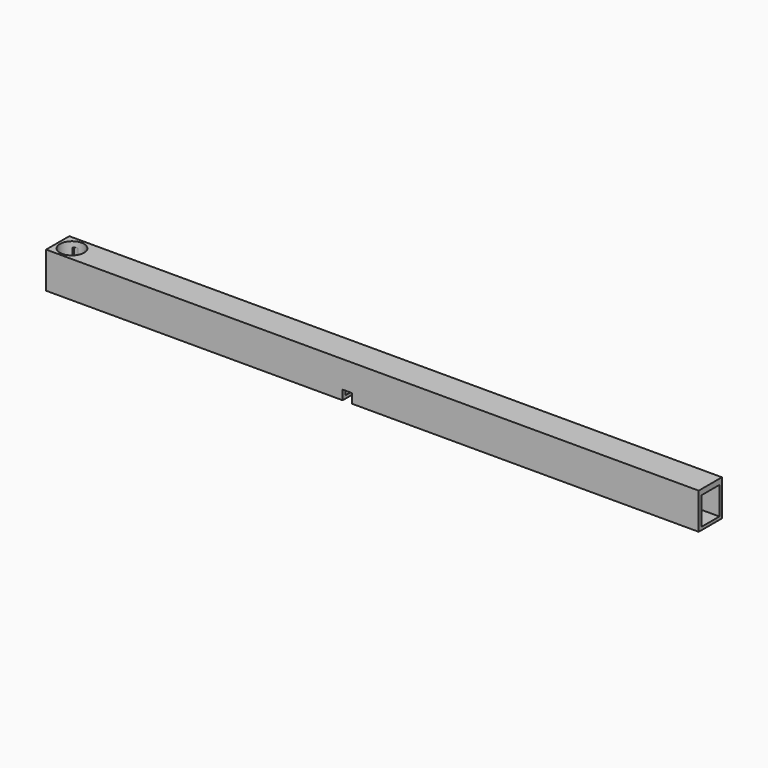
from build123d import *

# Parameters (mm, degrees)
F0_W     = 90
F0_H     = 4
F1_DEPTH = 5
F2_R     = 1.661067913
F3_DEPTH = 3.5
F6_W     = 1.3
F6_H     = 4
F7_DEPTH = 1.3
F8_W     = 3.1040143222
F8_H     = 3.8397812168
F9_DEPTH = 89


# Not quite as in the source:
# - the program builds the solid bodies; features that only make, move or delete a surface that nothing else refers to are left out


with BuildPart() as f1:
    # F0 (on Top) → F1 (new body)
    with BuildSketch(Plane.XY):
        with Locations((9.9665279686, 16.8302931339)):
            Rectangle(F0_W, F0_H)
    extrude(amount=F1_DEPTH)

    # F2 (on face) → F3 (cut)
    with BuildSketch(Plane.XY.offset(5)):
        with Locations((-33.0299064517, 16.7948473245)):
            Circle(F2_R)
    extrude(amount=-F3_DEPTH, mode=Mode.SUBTRACT)

    # F6 (on face) → F7 (cut)
    with BuildSketch(Plane(origin=(0, 0, 0), x_dir=(1, 0, 0), z_dir=(0, 0, -1))):
        with Locations((6.5131389402, -16.8302931339)):
            Rectangle(F6_W, F6_H)
    extrude(amount=-F7_DEPTH, mode=Mode.SUBTRACT)

    # F8 (on face) → F9 (cut)
    with BuildSketch(Plane.YZ.offset(54.9665279686)):
        with Locations((16.8456220999, 2.3313869315)):
            Rectangle(F8_W, F8_H)
    extrude(amount=-F9_DEPTH, mode=Mode.SUBTRACT)


solid = f1.part
